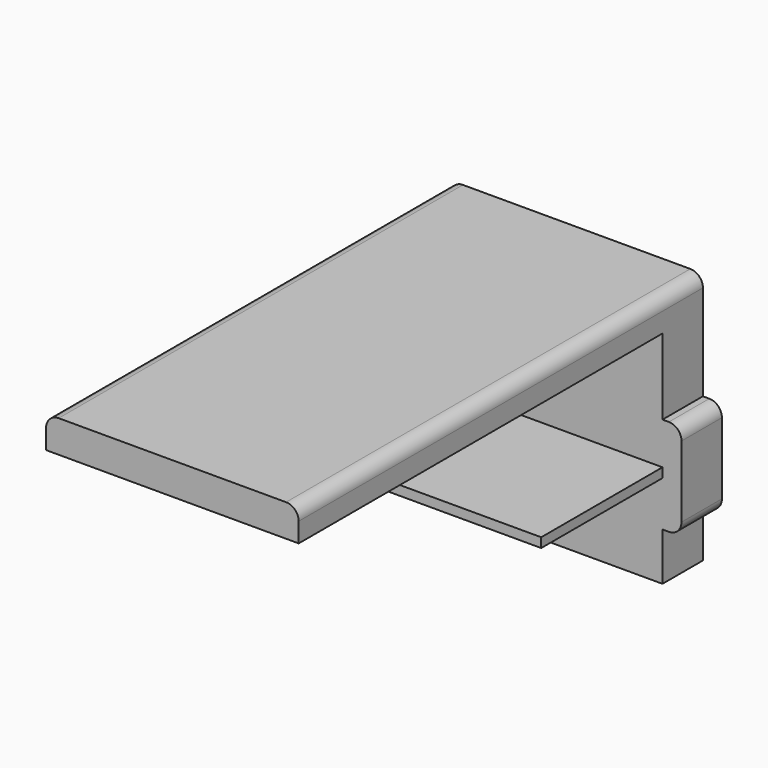
from build123d import *

# Parameters (mm, degrees)
F1_DEPTH  = 12.7
F0_W      = 63.5
F0_H      = 4.7856457531
F2_DEPTH  = 101.6
F3_DEPTH  = 254
F1_FACE_W = 127
F1_FACE_H = 46.801686123
F4_DEPTH  = 2.54
F6_DEPTH  = 25.4


# Not quite as in the source:
# - a feature of the source that left no trace in its solid (it failed there, or was rolled back) is left out


with BuildPart() as f1:
    # F0 (on Front) → F1 (new body)
    with BuildSketch(Plane.XZ):
        Polygon((6.9482082725, -25.8761684795), (-56.5517917275, -25.8761684795), (-56.5517917275, -47.4115650554), (-56.5517917275, -72.6778546025), (6.9482082725, -72.6778546025), align=None)
        Polygon((70.4482082725, -25.8761684795), (6.9482082725, -25.8761684795), (6.9482082725, -72.6778546025), (70.4482082725, -72.6778546025), (70.4482082725, -48.604208976), align=None)
    extrude(amount=F1_DEPTH)

    # F0 (on Front) → F2 (join)
    with BuildSketch(Plane.XZ):
        with Locations((-24.8017917275, -23.4833456029)):
            Rectangle(F0_W, F0_H)
        with Locations((38.6982082725, -23.4833456029)):
            Rectangle(F0_W, F0_H)
    extrude(amount=F2_DEPTH)

    # F0 (on Front) + F1_face (on face) → F4 (join)
    with BuildSketch(Plane.XZ):
        with BuildLine():
            Line((73.6600043416, 0), (70.4482082725, 0))
            Line((70.4482082725, 0), (70.4482082725, -21.0905227264))
            Line((70.4482082725, -21.0905227264), (70.4482082725, -25.8761684795))
            Line((70.4482082725, -25.8761684795), (70.4482082725, -48.604208976))
            Line((70.4482082725, -48.604208976), (73.6600043416, -48.604208976))
            ThreePointArc((73.6600043416, -48.604208976), (78.1501324021, -46.7443370366), (80.0100043416, -42.254208976))
            Line((80.0100043416, -42.254208976), (80.0100043416, -6.35))
            ThreePointArc((80.0100043416, -6.35), (78.1501324021, -1.8598719395), (73.6600043416, 0))
        make_face()
        with BuildLine():
            Line((-56.5517917275, -21.0905227264), (-56.5517917275, 0))
            Line((-56.5517917275, 0), (-61.3967882633, 0))
            ThreePointArc((-61.3967882633, 0), (-65.8869163239, -1.8598719395), (-67.7467882633, -6.35))
            Line((-67.7467882633, -6.35), (-67.7467882633, -41.0615650554))
            ThreePointArc((-67.7467882633, -41.0615650554), (-65.8869163239, -45.551693116), (-61.3967882633, -47.4115650554))
            Line((-61.3967882633, -47.4115650554), (-56.5517917275, -47.4115650554))
            Line((-56.5517917275, -47.4115650554), (-56.5517917275, -25.8761684795))
            Line((-56.5517917275, -25.8761684795), (-56.5517917275, -21.0905227264))
        make_face()
    with BuildSketch(Plane(origin=(6.9482082725, -12.7, -49.277011541), x_dir=(1, 0, 0), z_dir=(0, -1, 0))):
        Rectangle(F1_FACE_W, F1_FACE_H)
    extrude(amount=F4_DEPTH)



with BuildPart() as f3:
    # F0 (on Front) → F3 (new body)
    with BuildSketch(Plane.XZ):
        with BuildLine():
            ThreePointArc((-50.2017917275, 54.3221453975), (-54.6919197881, 52.462273458), (-56.5517917275, 47.9721453975))
            Line((-56.5517917275, 47.9721453975), (-56.5517917275, 38.1318327586))
            Line((-56.5517917275, 38.1318327586), (70.4482082725, 38.1318327586))
            Line((70.4482082725, 38.1318327586), (70.4482082725, 47.9721453975))
            ThreePointArc((70.4482082725, 47.9721453975), (68.588336333, 52.462273458), (64.0982082725, 54.3221453975))
            Line((64.0982082725, 54.3221453975), (-50.2017917275, 54.3221453975))
        make_face()
    extrude(amount=F3_DEPTH)


with BuildPart() as f1_1:
    add(f1.part)

    add(f3.part)  # F6 merges F3
    # F0 (on Front) → F6 (join)
    with BuildSketch(Plane.XZ):
        with BuildLine():
            ThreePointArc((-50.2017917275, 54.3221453975), (-54.6919197881, 52.462273458), (-56.5517917275, 47.9721453975))
            Line((-56.5517917275, 47.9721453975), (-56.5517917275, 38.1318327586))
            Line((-56.5517917275, 38.1318327586), (70.4482082725, 38.1318327586))
            Line((70.4482082725, 38.1318327586), (70.4482082725, 47.9721453975))
            ThreePointArc((70.4482082725, 47.9721453975), (68.588336333, 52.462273458), (64.0982082725, 54.3221453975))
            Line((64.0982082725, 54.3221453975), (-50.2017917275, 54.3221453975))
        make_face()
        Polygon((70.4482082725, 38.1318327586), (-56.5517917275, 38.1318327586), (-56.5517917275, 0), (-56.5517917275, -21.0905227264), (6.9482082725, -21.0905227264), (70.4482082725, -21.0905227264), (70.4482082725, 0), align=None)
        with BuildLine():
            Line((-56.5517917275, -21.0905227264), (-56.5517917275, 0))
            Line((-56.5517917275, 0), (-61.3967882633, 0))
            ThreePointArc((-61.3967882633, 0), (-65.8869163239, -1.8598719395), (-67.7467882633, -6.35))
            Line((-67.7467882633, -6.35), (-67.7467882633, -41.0615650554))
            ThreePointArc((-67.7467882633, -41.0615650554), (-65.8869163239, -45.551693116), (-61.3967882633, -47.4115650554))
            Line((-61.3967882633, -47.4115650554), (-56.5517917275, -47.4115650554))
            Line((-56.5517917275, -47.4115650554), (-56.5517917275, -25.8761684795))
            Line((-56.5517917275, -25.8761684795), (-56.5517917275, -21.0905227264))
        make_face()
        with BuildLine():
            Line((73.6600043416, 0), (70.4482082725, 0))
            Line((70.4482082725, 0), (70.4482082725, -21.0905227264))
            Line((70.4482082725, -21.0905227264), (70.4482082725, -25.8761684795))
            Line((70.4482082725, -25.8761684795), (70.4482082725, -48.604208976))
            Line((70.4482082725, -48.604208976), (73.6600043416, -48.604208976))
            ThreePointArc((73.6600043416, -48.604208976), (78.1501324021, -46.7443370366), (80.0100043416, -42.254208976))
            Line((80.0100043416, -42.254208976), (80.0100043416, -6.35))
            ThreePointArc((80.0100043416, -6.35), (78.1501324021, -1.8598719395), (73.6600043416, 0))
        make_face()
        Polygon((6.9482082725, -25.8761684795), (-56.5517917275, -25.8761684795), (-56.5517917275, -47.4115650554), (-56.5517917275, -72.6778546025), (6.9482082725, -72.6778546025), align=None)
        Polygon((70.4482082725, -25.8761684795), (6.9482082725, -25.8761684795), (6.9482082725, -72.6778546025), (70.4482082725, -72.6778546025), (70.4482082725, -48.604208976), align=None)
    extrude(amount=F6_DEPTH)


solid = f1_1.part
